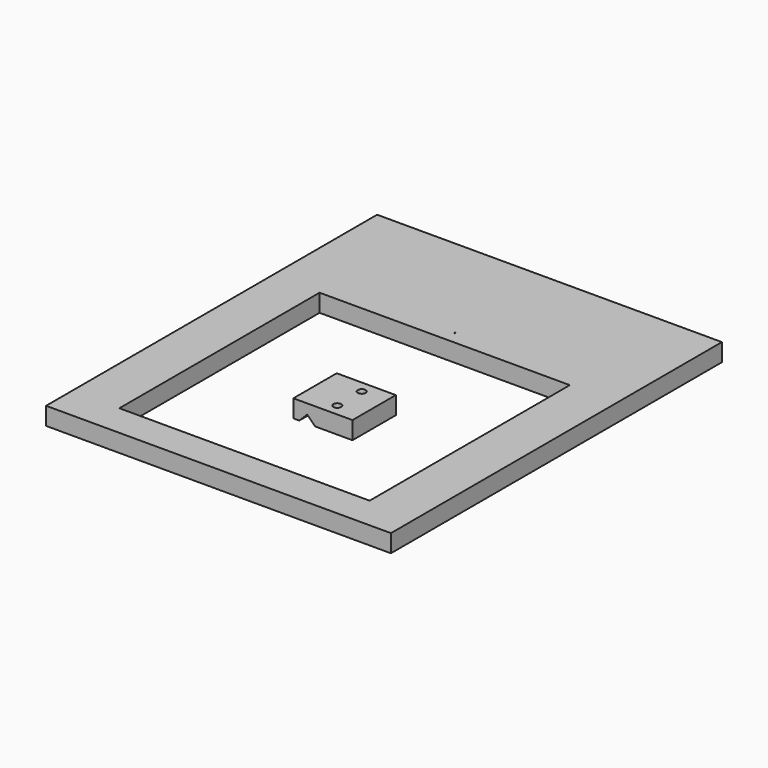
from build123d import *

# Parameters (mm, degrees)
F0_W     = 350
F0_H     = 420
F0_W_2   = 254
F0_H_2   = 254
F1_DEPTH = 18
F2_D     = 1
F3_W     = 60
F3_H     = 55
F4_DEPTH = 18
F5_D     = 8
F7_DEPTH = 287.501


with BuildPart() as f1:
    # F0 (on Top) → F1 (new body)
    with BuildSketch(Plane.XY):
        with Locations((0, 50)):
            Rectangle(F0_W, F0_H)
        Rectangle(F0_W_2, F0_H_2, mode=Mode.SUBTRACT)
    extrude(amount=F1_DEPTH)

    # F2 (through all)
    with Locations(Plane(origin=(0, 0, 0), x_dir=(1, 0, 0), z_dir=(0, 0, -1))):
        with Locations((0, -140)):
            Hole(F2_D / 2)


with BuildPart() as f4:
    # F3 (on Top) → F4 (new body)
    with BuildSketch(Plane.XY):
        Rectangle(F3_W, F3_H)
    extrude(amount=F4_DEPTH)

    # F5 (through all)
    with Locations(Plane(origin=(0, 0, 0), x_dir=(1, 0, 0), z_dir=(0, 0, -1))):
        with Locations((5, -15.5), (5, 15.5)):
            Hole(F5_D / 2)

    # F6 (on face) → F7 (cut, through all)
    with BuildSketch(Plane.XZ.offset(27.5)):
        Polygon((-8, 0), (-16, 8), (-24, 0), align=None)
    extrude(amount=-F7_DEPTH, mode=Mode.SUBTRACT)


solid = Compound([f1.part, f4.part])
